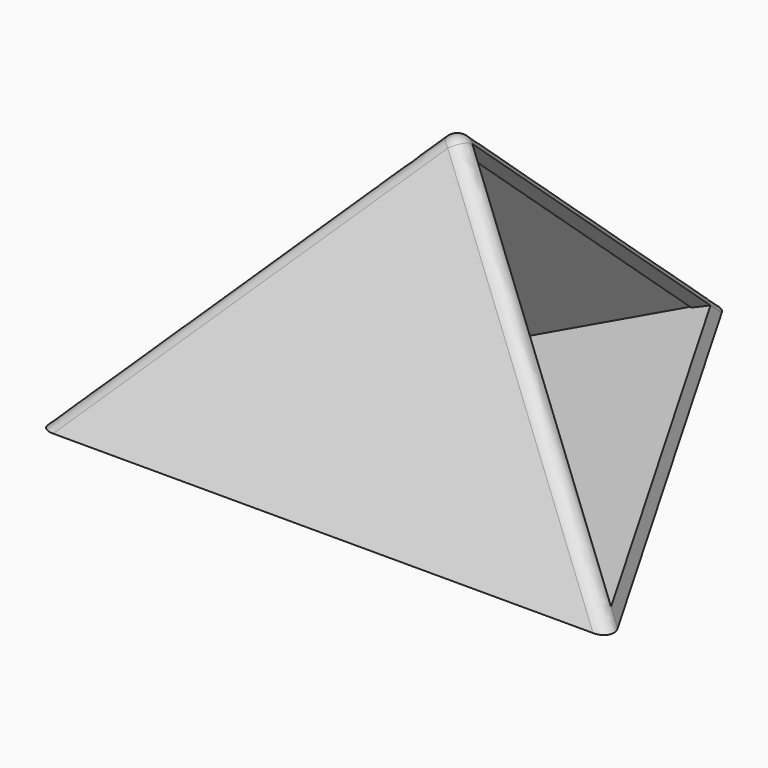
from build123d import *

# Parameters (mm, degrees)
F4_R = 3.5
F5_T = 3.175


# Not quite as in the source:
# - a shell that OpenCascade refuses in one call is made with other operations: the cavity is built on its own and cut out


with BuildPart() as f3:
    # F0 (on Top) → F3 section 0
    with BuildSketch(Plane.XY, mode=Mode.PRIVATE) as f3_s0:
        Polygon((74.6125, -43.0775469599), (0, 86.1550939198), (-74.6125, -43.0775469599), align=None)
    loft([f3_s0.sketch, Vertex(0, 0, 76.2)])

    # F4
    f4_edges = [f3.edges().sort_by_distance(p)[0] for p in [
        (37.30625, -21.538773, 38.1),
        (-37.30625, -21.538773, 38.1),
        (0, 43.077547, 38.1),
    ]]
    fillet(f4_edges, radius=F4_R)

    # F5: shell of thickness 3.175, made by hand


with BuildPart() as f5_core1:
    # F5_t2: copy of F3
    add(f3.part)

    # the walls: a layer under each face that stays
    f5_faces = [f5_core1.faces().sort_by_distance(p)[0] for p in [
        (0, -23.0621900868, 35.4052238664),
        (17.458808121, -10.0798475684, 0),
        (-37.1159888559, -21.4289261572, 35.8548532751),
        (37.1159888559, -21.4289261572, 35.8548532751),
        (-19.9724424821, 11.5310950434, 35.4052238664),
        (0, 42.8578523144, 35.8548532751),
        (-0.5010139072, 0.2892605142, 72.5398619822),
    ]]
    thicken(f5_faces, amount=-F5_T, mode=Mode.SUBTRACT)


with BuildPart() as f3_1:
    add(f3.part)

    # what is left inside the walls is the cavity
    f5_cavity = [f5_core1.part.solids().sort_by_distance(p)[0] for p in [
        (1.753709, 1.221373, 3.20675),
    ]]
    add(f5_cavity, mode=Mode.SUBTRACT)


solid = f3_1.part
